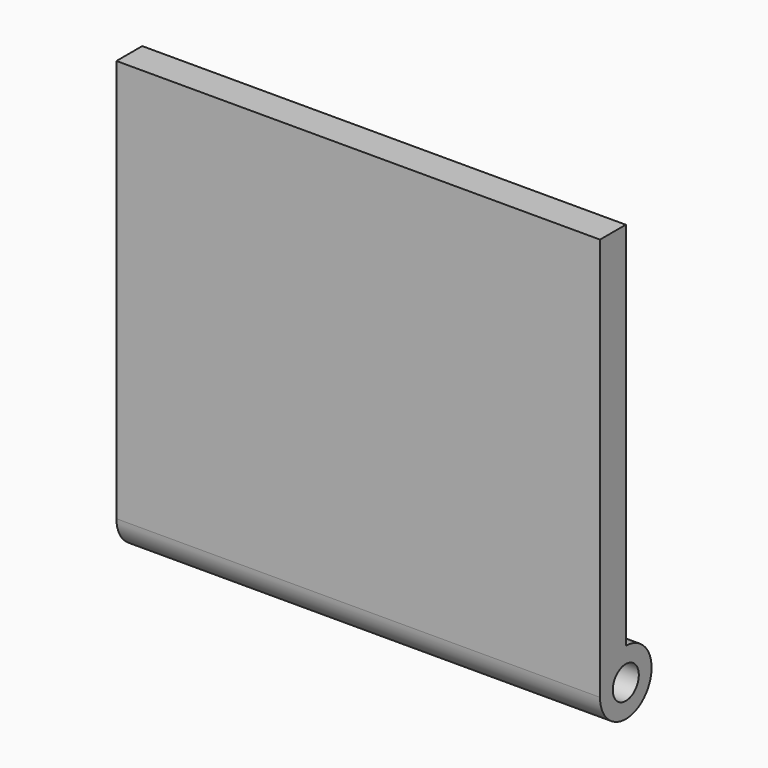
from build123d import *

# Parameters (mm, degrees)
F2_DEPTH = 30


# Not quite as in the source:
# - a feature of the source that left no trace in its solid (it failed there, or was rolled back) is left out


with BuildPart() as f2:
    # F1 (on Right) → F2 (new body)
    with BuildSketch(Plane.YZ):
        with BuildLine():
            Line((0, 25), (0, 0))
            ThreePointArc((0, 0), (3.4142135624, -1.4142135624), (2, 2))
            Line((2, 2), (2, 25))
            Line((2, 25), (0, 25))
        make_face()
        with BuildLine():
            ThreePointArc((3.01, 0), (2, -1.01), (0.99, 0))
            ThreePointArc((0.99, 0), (2, 1.01), (3.01, 0))
        make_face(mode=Mode.SUBTRACT)
    extrude(amount=F2_DEPTH)


solid = f2.part
